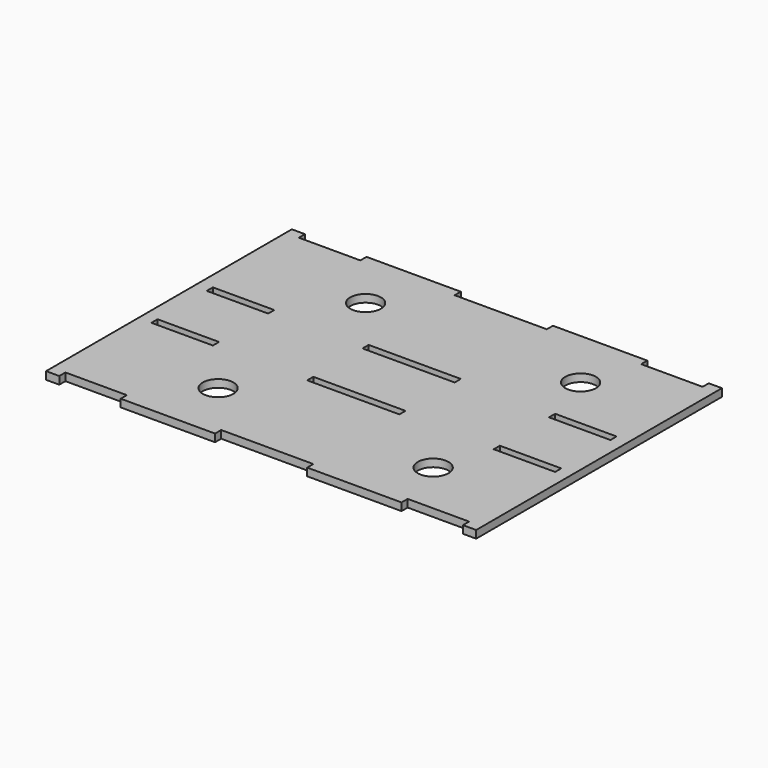
from build123d import *

# Parameters (mm, degrees)
F0_R     = 6.35
F0_W     = 25.4
F0_H     = 3.175
F0_W_2   = 38.1
F1_DEPTH = 3.175


# Not quite as in the source:
# - a feature names something its author has since deleted; it is built from what else it names


with BuildPart() as f1:
    # F0 (on Top) → F1 (new body)
    with BuildSketch(Plane.XY):
        Polygon((-70.7512, 63.5), (-76.2, 63.5), (-76.2, -63.5), (-70.7512, -63.5), (-70.7512, -60.325), (-45.3512, -60.325), (-45.3512, -63.5), (-6.35, -63.5), (-6.35, -60.325), (31.75, -60.325), (31.75, -63.5), (70.7512, -63.5), (70.7512, -60.325), (96.1512, -60.325), (96.1512, -63.5), (101.6, -63.5), (101.6, 63.5), (96.1512, 63.5), (96.1512, 60.325), (70.7512, 60.325), (70.7512, 63.5), (31.75, 63.5), (31.75, 60.325), (-6.35, 60.325), (-6.35, 63.5), (-45.3512, 63.5), (-45.3512, 60.325), (-70.7512, 60.325), align=None)
        with Locations((-25.4, -38.1)):
            Circle(F0_R, mode=Mode.SUBTRACT)
        with Locations((-58.0512, -14.2875)):
            Rectangle(F0_W, F0_H, mode=Mode.SUBTRACT)
        with Locations((63.5, -38.1)):
            Circle(F0_R, mode=Mode.SUBTRACT)
        with Locations((12.7, -14.2875)):
            Rectangle(F0_W_2, F0_H, mode=Mode.SUBTRACT)
        with Locations((83.4512, -14.2875)):
            Rectangle(F0_W, F0_H, mode=Mode.SUBTRACT)
        with Locations((-58.0512, 14.2875)):
            Rectangle(F0_W, F0_H, mode=Mode.SUBTRACT)
        with Locations((-25.4, 38.1)):
            Circle(F0_R, mode=Mode.SUBTRACT)
        with Locations((12.7, 14.2875)):
            Rectangle(F0_W_2, F0_H, mode=Mode.SUBTRACT)
        with Locations((83.4512, 14.2875)):
            Rectangle(F0_W, F0_H, mode=Mode.SUBTRACT)
        with Locations((63.5, 38.1)):
            Circle(F0_R, mode=Mode.SUBTRACT)
    extrude(amount=F1_DEPTH)


solid = f1.part
